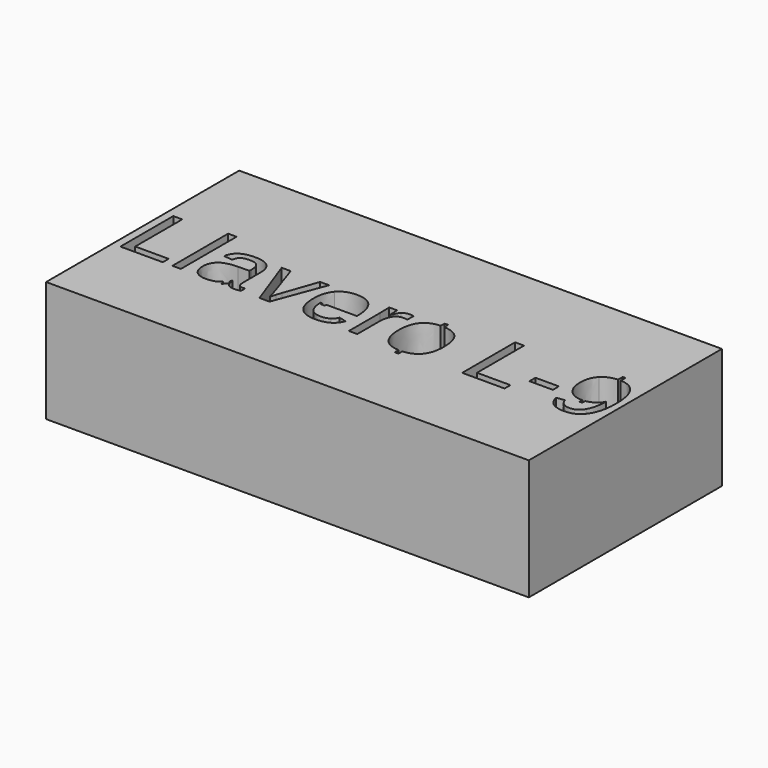
from build123d import *

# Parameters (mm, degrees)
F0_W     = 100
F0_H     = 50
F0_W_2   = 1.7507852101
F0_H_2   = 14.422987219
F0_W_3   = 4.8605280343
F0_H_3   = 1.5548714121
F1_DEPTH = 25


with BuildPart() as f1:
    # F0 (on Top) → F1 (new body)
    with BuildSketch(Plane.XY):
        with Locations((50, -25)):
            Rectangle(F0_W, F0_H)
        Polygon((10.4083092328, -32.793873014), (1.6326149827, -32.793873014), (1.6326149827, -19.1016753587), (3.4891314488, -19.1016753587), (3.4891314488, -31.2763185157), (10.4083092328, -31.2763185157), align=None, mode=Mode.SUBTRACT)
        with Locations((13.2832664739, -25.5823794045)):
            Rectangle(F0_W_2, F0_H_2, mode=Mode.SUBTRACT)
        with BuildLine():
            add(Edge.make_bspline(
                [(23.2359983829, -30.7818694067), (23.1275453776, -30.9766831384), (23.0134175895, -31.1530943602)],
                knots=[0, 0, 0, 0.1614594117, 0.1614594117, 0.1614594117], degree=2))
            Line((23.0134175895, -31.1530943602), (23.3730170876, -31.9282598794))
            Line((23.3730170876, -31.9282598794), (22.5588716567, -32.793873014))
            Line((22.5588716567, -32.793873014), (22.2831973701, -32.0407349492))
            add(Edge.make_bspline(
                [(22.2831973701, -32.0407349492), (21.9929725637, -32.310067596), (21.6749074852, -32.4891182172)],
                knots=[0.6423769674, 0.6423769674, 0.6423769674, 1, 1, 1], degree=2))
            add(Edge.make_bspline(
                [(21.6749074852, -32.4891182172), (20.7855210374, -32.9897868119), (19.5136362223, -32.9897868119)],
                knots=[0, 0, 0, 1, 1, 1], degree=2))
            add(Edge.make_bspline(
                [(19.5136362223, -32.9897868119), (17.9276673819, -32.9897868119), (17.1315732189, -32.1532659922)],
                knots=[0, 0, 0, 1, 1, 1], degree=2))
            add(Edge.make_bspline(
                [(17.1315732189, -32.1532659922), (16.3354790559, -31.3167451724), (16.3354790559, -29.8582757879)],
                knots=[0, 0, 0, 1, 1, 1], degree=2))
            add(Edge.make_bspline(
                [(16.3354790559, -29.8582757879), (16.3354790559, -28.2256608051), (17.4098952017, -27.3518230715)],
                knots=[0, 0, 0, 1, 1, 1], degree=2))
            add(Edge.make_bspline(
                [(17.4098952017, -27.3518230715), (18.4843113475, -26.4779853379), (20.8725938365, -26.4189002242)],
                knots=[0, 0, 0, 1, 1, 1], degree=2))
            Line((20.8725938365, -26.4189002242), (23.2359983829, -26.3784735675))
            Line((23.2359983829, -26.3784735675), (23.2359983829, -25.8062808878))
            add(Edge.make_bspline(
                [(23.2359983829, -25.8062808878), (23.2359983829, -24.5250668442), (22.6917933887, -23.9699777501)],
                knots=[0, 0, 0, 1, 1, 1], degree=2))
            add(Edge.make_bspline(
                [(22.6917933887, -23.9699777501), (22.1475883944, -23.414888656), (20.9814348353, -23.414888656)],
                knots=[0, 0, 0, 1, 1, 1], degree=2))
            add(Edge.make_bspline(
                [(20.9814348353, -23.414888656), (19.8059520478, -23.414888656), (19.271076282, -23.8144906089)],
                knots=[0, 0, 0, 1, 1, 1], degree=2))
            add(Edge.make_bspline(
                [(19.271076282, -23.8144906089), (18.7362005162, -24.2140925618), (18.6273595174, -25.0879302954)],
                knots=[0, 0, 0, 1, 1, 1], degree=2))
            Line((18.6273595174, -25.0879302954), (16.8019404795, -24.9231139257))
            add(Edge.make_bspline(
                [(16.8019404795, -24.9231139257), (17.2497434462, -22.0839187272), (21.0187517492, -22.0839187272)],
                knots=[0, 0, 0, 1, 1, 1], degree=2))
            add(Edge.make_bspline(
                [(21.0187517492, -22.0839187272), (23.0027676711, -22.0839187272), (24.0025499891, -22.9935185033)],
                knots=[0, 0, 0, 1, 1, 1], degree=2))
            add(Edge.make_bspline(
                [(24.0025499891, -22.9935185033), (25.0023323071, -23.9031182794), (25.0023323071, -25.6228060612)],
                knots=[0, 0, 0, 1, 1, 1], degree=2))
            Line((25.0023323071, -25.6228060612), (25.0023323071, -30.1505916133))
            add(Edge.make_bspline(
                [(25.0023323071, -30.1505916133), (25.0023323071, -30.9280273194), (25.2075753335, -31.3214097867)],
                knots=[0, 0, 0, 1, 1, 1], degree=2))
            add(Edge.make_bspline(
                [(25.2075753335, -31.3214097867), (25.4128183599, -31.7147922539), (25.9850110396, -31.7147922539)],
                knots=[0, 0, 0, 1, 1, 1], degree=2))
            add(Edge.make_bspline(
                [(25.9850110396, -31.7147922539), (26.2369002084, -31.7147922539), (26.5572037193, -31.6463779118)],
                knots=[0, 0, 0, 1, 1, 1], degree=2))
            Line((26.5572037193, -31.6463779118), (26.5572037193, -32.7347879003))
            add(Edge.make_bspline(
                [(26.5572037193, -32.7347879003), (25.8979382405, -32.8902750415), (25.2075753335, -32.8902750415)],
                knots=[0, 0, 0, 1, 1, 1], degree=2))
            add(Edge.make_bspline(
                [(25.2075753335, -32.8902750415), (24.2373355723, -32.8902750415), (23.7941972199, -32.3802772183)],
                knots=[0, 0, 0, 1, 1, 1], degree=2))
            add(Edge.make_bspline(
                [(23.7941972199, -32.3802772183), (23.3510588674, -31.8702793952), (23.2919737538, -30.7818694067)],
                knots=[0, 0, 0, 1, 1, 1], degree=2))
            Line((23.2919737538, -30.7818694067), (23.2359983829, -30.7818694067))
        make_face(mode=Mode.SUBTRACT)
        with BuildLine():
            Line((36.4399664148, -22.2798325251), (32.5154709706, -32.793873014))
            Line((32.5154709706, -32.793873014), (30.4443822496, -32.793873014))
            Line((30.4443822496, -32.793873014), (26.6256180614, -22.2798325251))
            Line((26.6256180614, -22.2798325251), (28.4914637559, -22.2798325251))
            Line((28.4914637559, -22.2798325251), (30.8051124172, -29.1212667385))
            add(Edge.make_bspline(
                [(30.8051124172, -29.1212667385), (30.9295021302, -29.5099845915), (31.4737071244, -31.4224764285)],
                knots=[0, 0, 0, 1, 1, 1], degree=2))
            Line((31.4737071244, -31.4224764285), (31.8157788351, -30.2874202976))
            Line((31.8157788351, -30.2874202976), (32.1951674597, -29.1399251955))
            Line((32.1951674597, -29.1399251955), (34.5834499487, -22.2798325251))
            Line((34.5834499487, -22.2798325251), (36.4399664148, -22.2798325251))
        make_face(mode=Mode.SUBTRACT)
        with BuildLine():
            Line((39.5392887294, -28.3074099571), (39.5392887294, -27.9053572942))
            Line((39.5392887294, -27.9053572942), (39.1920888143, -27.9053572942))
            add(Edge.make_bspline(
                [(39.1920888143, -27.9053572942), (39.1920888143, -29.7121178751), (39.9399819635, -30.6947966076)],
                knots=[0, 0, 0, 1, 1, 1], degree=2))
            add(Edge.make_bspline(
                [(39.9399819635, -30.6947966076), (40.6878751127, -31.6774753401), (42.1245762975, -31.6774753401)],
                knots=[0, 0, 0, 1, 1, 1], degree=2))
            add(Edge.make_bspline(
                [(42.1245762975, -31.6774753401), (43.2627421712, -31.6774753401), (43.948440464, -31.2203431449)],
                knots=[0, 0, 0, 1, 1, 1], degree=2))
            add(Edge.make_bspline(
                [(43.948440464, -31.2203431449), (44.6341387567, -30.7632109497), (44.876698697, -30.0635188143)],
                knots=[0, 0, 0, 1, 1, 1], degree=2))
            Line((44.876698697, -30.0635188143), (46.4098019094, -30.4988828097))
            add(Edge.make_bspline(
                [(46.4098019094, -30.4988828097), (45.4675498336, -32.9897868119), (42.1245762975, -32.9897868119)],
                knots=[0, 0, 0, 1, 1, 1], degree=2))
            add(Edge.make_bspline(
                [(42.1245762975, -32.9897868119), (39.7922691793, -32.9897868119), (38.5732499922, -31.5997317694)],
                knots=[0, 0, 0, 1, 1, 1], degree=2))
            add(Edge.make_bspline(
                [(38.5732499922, -31.5997317694), (37.3542308051, -30.209676727), (37.3542308051, -27.466883556)],
                knots=[0, 0, 0, 1, 1, 1], degree=2))
            add(Edge.make_bspline(
                [(37.3542308051, -27.466883556), (37.3542308051, -24.8640288121), (38.5732499922, -23.4739737696)],
                knots=[0, 0, 0, 1, 1, 1], degree=2))
            add(Edge.make_bspline(
                [(38.5732499922, -23.4739737696), (39.7922691793, -22.0839187272), (42.0561619554, -22.0839187272)],
                knots=[0, 0, 0, 1, 1, 1], degree=2))
            add(Edge.make_bspline(
                [(42.0561619554, -22.0839187272), (46.6927885064, -22.0839187272), (46.6927885064, -27.6721265824)],
                knots=[0, 0, 0, 1, 1, 1], degree=2))
            Line((46.6927885064, -27.6721265824), (46.6927885064, -27.9053572942))
            Line((46.6927885064, -27.9053572942), (40.3838679194, -27.9053572942))
            Line((40.3838679194, -27.9053572942), (40.3838679194, -28.3074099571))
            Line((40.3838679194, -28.3074099571), (39.5392887294, -28.3074099571))
        make_face(mode=Mode.SUBTRACT)
        with BuildLine():
            Line((50.7043567497, -32.793873014), (48.9566812825, -32.793873014))
            Line((48.9566812825, -32.793873014), (48.9566812825, -24.7272001278))
            add(Edge.make_bspline(
                [(48.9566812825, -24.7272001278), (48.9566812825, -23.6201316824), (48.8975961688, -22.2798325251)],
                knots=[0, 0, 0, 1, 1, 1], degree=2))
            Line((48.8975961688, -22.2798325251), (50.5488696085, -22.2798325251))
            add(Edge.make_bspline(
                [(50.5488696085, -22.2798325251), (50.6266131791, -24.0679346491), (50.6266131791, -24.4255550739)],
                knots=[0, 0, 0, 1, 1, 1], degree=2))
            Line((50.6266131791, -24.4255550739), (50.6670398358, -24.4255550739))
            add(Edge.make_bspline(
                [(50.6670398358, -24.4255550739), (51.0837453743, -23.0759266881), (51.6279503685, -22.5799227077)],
                knots=[0, 0, 0, 1, 1, 1], degree=2))
            add(Edge.make_bspline(
                [(51.6279503685, -22.5799227077), (52.1721553628, -22.0839187272), (53.1641633237, -22.0839187272)],
                knots=[0, 0, 0, 1, 1, 1], degree=2))
            add(Edge.make_bspline(
                [(53.1641633237, -22.0839187272), (53.51245452, -22.0839187272), (53.8731846876, -22.1803207547)],
                knots=[0, 0, 0, 1, 1, 1], degree=2))
            Line((53.8731846876, -22.1803207547), (53.8731846876, -23.7849480521))
            add(Edge.make_bspline(
                [(53.8731846876, -23.7849480521), (53.5248934913, -23.6885460245), (52.9402618403, -23.6885460245)],
                knots=[0, 0, 0, 1, 1, 1], degree=2))
            add(Edge.make_bspline(
                [(52.9402618403, -23.6885460245), (51.8518518519, -23.6885460245), (51.2781043008, -24.626133486)],
                knots=[0, 0, 0, 1, 1, 1], degree=2))
            add(Edge.make_bspline(
                [(51.2781043008, -24.626133486), (50.7043567497, -25.5637209475), (50.7043567497, -27.3113964148)],
                knots=[0, 0, 0, 1, 1, 1], degree=2))
            Line((50.7043567497, -27.3113964148), (50.7043567497, -32.793873014))
        make_face(mode=Mode.SUBTRACT)
        with BuildLine():
            Line((59.4151429832, -22.091073404), (59.4151429832, -21.1587541808))
            Line((59.4151429832, -21.1587541808), (60.178603977, -21.0526138544))
            Line((60.178603977, -21.0526138544), (60.178603977, -22.0948970541))
            add(Edge.make_bspline(
                [(60.178603977, -22.0948970541), (62.264199739, -22.2045860937), (63.298815188, -23.4102240417)],
                knots=[0.0909800822, 0.0909800822, 0.0909800822, 1, 1, 1], degree=2))
            add(Edge.make_bspline(
                [(63.298815188, -23.4102240417), (64.4369810617, -24.7365293563), (64.4369810617, -27.5259686697)],
                knots=[0, 0, 0, 1, 1, 1], degree=2))
            add(Edge.make_bspline(
                [(64.4369810617, -27.5259686697), (64.4369810617, -30.2874202976), (63.2210716174, -31.6386035548)],
                knots=[0, 0, 0, 1, 1, 1], degree=2))
            add(Edge.make_bspline(
                [(63.2210716174, -31.6386035548), (62.1358349186, -32.8445763057), (60.178603977, -32.9741811633)],
                knots=[0, 0, 0, 0.8925308574, 0.8925308574, 0.8925308574], degree=2))
            Line((60.178603977, -32.9741811633), (60.178603977, -33.9884571731))
            Line((60.178603977, -33.9884571731), (59.4151429832, -33.9884571731))
            Line((59.4151429832, -33.9884571731), (59.4151429832, -32.9844581394))
            add(Edge.make_bspline(
                [(59.4151429832, -32.9844581394), (57.3179278624, -32.9032420138), (56.2148210343, -31.5841830553)],
                knots=[0.0615712627, 0.0615712627, 0.0615712627, 1, 1, 1], degree=2))
            add(Edge.make_bspline(
                [(56.2148210343, -31.5841830553), (55.0393382467, -30.1785792988), (55.0393382467, -27.5259686697)],
                knots=[0, 0, 0, 1, 1, 1], degree=2))
            add(Edge.make_bspline(
                [(55.0393382467, -27.5259686697), (55.0393382467, -22.2812410735), (59.4151429832, -22.091073404)],
                knots=[0, 0, 0, 0.9637411732, 0.9637411732, 0.9637411732], degree=2))
        make_face(mode=Mode.SUBTRACT)
        Polygon((81.2078241129, -32.793873014), (72.4321298629, -32.793873014), (72.4321298629, -19.1016753587), (74.2886463289, -19.1016753587), (74.2886463289, -31.2763185157), (81.2078241129, -31.2763185157), align=None, mode=Mode.SUBTRACT)
        with Locations((85.1805205709, -27.5073102127)):
            Rectangle(F0_W_3, F0_H_3, mode=Mode.SUBTRACT)
        with BuildLine():
            Line((93.6008840799, -18.9067042401), (93.6008840799, -17.7203528583))
            Line((93.6008840799, -17.7203528583), (94.1538438201, -17.6602434367))
            Line((94.1538438201, -17.6602434367), (94.1538438201, -18.8987676682))
            add(Edge.make_bspline(
                [(94.1538438201, -18.8987676682), (96.3119832442, -18.9592868311), (97.4437913985, -20.5881324287)],
                knots=[0.0371546345, 0.0371546345, 0.0371546345, 1, 1, 1], degree=2))
            add(Edge.make_bspline(
                [(97.4437913985, -20.5881324287), (98.619274186, -22.2798325251), (98.619274186, -25.6694522036)],
                knots=[0, 0, 0, 1, 1, 1], degree=2))
            add(Edge.make_bspline(
                [(98.619274186, -25.6694522036), (98.619274186, -29.1990103091), (97.3318406568, -31.0943985605)],
                knots=[0, 0, 0, 1, 1, 1], degree=2))
            add(Edge.make_bspline(
                [(97.3318406568, -31.0943985605), (96.0444071275, -32.9897868119), (93.665453867, -32.9897868119)],
                knots=[0, 0, 0, 1, 1, 1], degree=2))
            add(Edge.make_bspline(
                [(93.665453867, -32.9897868119), (92.0608265696, -32.9897868119), (91.0936965513, -32.3134177476)],
                knots=[0, 0, 0, 1, 1, 1], degree=2))
            add(Edge.make_bspline(
                [(91.0936965513, -32.3134177476), (90.1265665329, -31.6370486833), (89.7098609945, -30.1319331564)],
                knots=[0, 0, 0, 1, 1, 1], degree=2))
            Line((89.7098609945, -30.1319331564), (91.3797928911, -29.8676050163))
            add(Edge.make_bspline(
                [(91.3797928911, -29.8676050163), (91.9053394284, -31.5779635697), (93.6934415524, -31.5779635697)],
                knots=[0, 0, 0, 1, 1, 1], degree=2))
            add(Edge.make_bspline(
                [(93.6934415524, -31.5779635697), (95.1985570793, -31.5779635697), (96.0257486706, -30.1785792988)],
                knots=[0, 0, 0, 1, 1, 1], degree=2))
            add(Edge.make_bspline(
                [(96.0257486706, -30.1785792988), (96.8529402618, -28.7791950278), (96.8902571757, -26.1856695124)],
                knots=[0, 0, 0, 1, 1, 1], degree=2))
            add(Edge.make_bspline(
                [(96.8902571757, -26.1856695124), (96.5015393227, -27.059507246), (95.5592872469, -27.5897183976)],
                knots=[0, 0, 0, 1, 1, 1], degree=2))
            add(Edge.make_bspline(
                [(95.5592872469, -27.5897183976), (94.9019666015, -27.9595968465), (94.1538438201, -28.0714458923)],
                knots=[0, 0, 0, 0.6976059404, 0.6976059404, 0.6976059404], degree=2))
            Line((94.1538438201, -28.0714458923), (94.1538438201, -28.8373995572))
            Line((94.1538438201, -28.8373995572), (93.6008840799, -28.8373995572))
            Line((93.6008840799, -28.8373995572), (93.6008840799, -28.1185976588))
            add(Edge.make_bspline(
                [(93.6008840799, -28.1185976588), (93.5447756531, -28.1199295491), (93.488198526, -28.1199295491)],
                knots=[0.9498801466, 0.9498801466, 0.9498801466, 1, 1, 1], degree=2))
            add(Edge.make_bspline(
                [(93.488198526, -28.1199295491), (91.6441210312, -28.1199295491), (90.5354977143, -26.855819091)],
                knots=[0, 0, 0, 1, 1, 1], degree=2))
            add(Edge.make_bspline(
                [(90.5354977143, -26.855819091), (89.4268743975, -25.591708633), (89.4268743975, -23.5019614551)],
                knots=[0, 0, 0, 1, 1, 1], degree=2))
            add(Edge.make_bspline(
                [(89.4268743975, -23.5019614551), (89.4268743975, -21.3562389063), (90.6318997419, -20.1263356193)],
                knots=[0, 0, 0, 1, 1, 1], degree=2))
            add(Edge.make_bspline(
                [(90.6318997419, -20.1263356193), (91.7268000016, -19.0088309671), (93.6008840799, -18.9067042401)],
                knots=[0, 0, 0, 0.9086118104, 0.9086118104, 0.9086118104], degree=2))
        make_face(mode=Mode.SUBTRACT)
    extrude(amount=F1_DEPTH)


solid = f1.part
